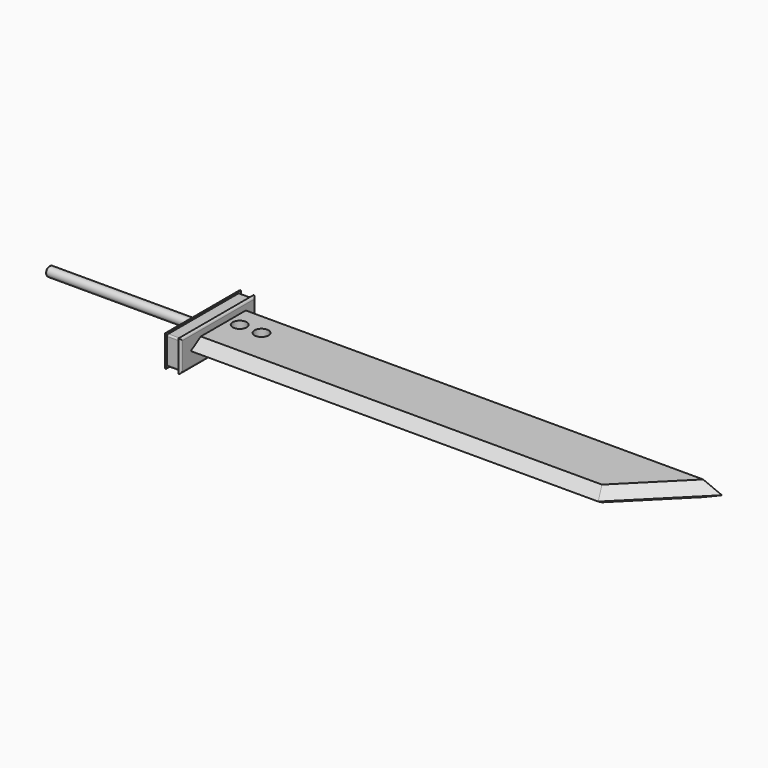
from build123d import *

# Parameters (mm, degrees)
F1_DEPTH    = 25
F2_T1_DEPTH = 1920.4823536212
F3_T1_DEPTH = 694.2958053538
F5_R        = 22.5
F6_DEPTH    = 100
F7_W        = 55
F7_H        = 300
F8_DEPTH    = 50
F9_R        = 7
F10_DEPTH   = 5
F11_DEPTH   = 5
F12_DEPTH   = 5
F13_DEPTH   = 5
F14_R       = 5
F15_W       = 500
F15_H       = 15
F17_R       = 5
F18_R       = 5


# Not quite as in the source:
# - a fillet or chamfer that OpenCascade refuses, or shapes differently, is made with other operations: its cross-section is extruded or revolved along the edge and cut away or added
# - a feature names something its author has since deleted; it is built from what else it names


with BuildPart() as f1:
    # F0 (on Top) → F1 (new body)
    with BuildSketch(Plane.XY):
        Polygon((1600, 0), (0, 0), (0, -300), (1300, -300), align=None)
    extrude(amount=F1_DEPTH)

    # F2: chamfer of 120 x 75 on 1 edges, made by hand

    # F2_s2 → F2_t1 (cut)
    with BuildSketch(Plane.YZ.offset(-310.2411768106)):
        Polygon((-300, -50), (-180, 25), (-300, 25), align=None)
    extrude(amount=F2_T1_DEPTH, mode=Mode.SUBTRACT)

    # F3: chamfer of 50 x 85 on 1 edges, made by hand

    # F3_s2 → F3_t1 (cut)
    with BuildSketch(Plane(origin=(464.5293639425, 464.5293639425, 0), x_dir=(0, 0, 1), z_dir=(0.7071067812, 0.7071067812, 0))):
        Polygon((-25, 1131.3708498985), (25, 1046.3708498985), (25, 1131.3708498985), align=None)
    extrude(amount=F3_T1_DEPTH, mode=Mode.SUBTRACT)

    # F4: F1 across face


with BuildPart() as f1_1:
    add(f1.part)
    add(f1.part.mirror(Plane(origin=(716.3583208568, -107.1792818856, 0), x_dir=(1, 0, 0), z_dir=(0, 0, -1))))

    # F5 (on face) → F6 (cut)
    with BuildSketch(Plane.XY.offset(25)):
        with Locations((52, -70)):
            Circle(F5_R)
        with Locations((122, -70)):
            Circle(F5_R)
    extrude(amount=-F6_DEPTH, mode=Mode.SUBTRACT)


with BuildPart() as f8:
    # F7 (on Top) → F8 (new body, symmetric)
    with BuildSketch(Plane.XY):
        with Locations((-11.9931862531, -110)):
            Rectangle(F7_W, F7_H)
    extrude(amount=F8_DEPTH, both=True)

    # F9
    f9_edges = [f8.edges().sort_by_distance(p)[0] for p in [
        (15.506814, -110, 50),
        (15.506814, -110, -50),
        (-39.493186, -110, 50),
        (-39.493186, -260, 0),
        (-39.493186, -110, -50),
        (-39.493186, 40, 0),
        (15.506814, -260, 0),
        (15.506814, 40, 0),
    ]]
    fillet(f9_edges, radius=F9_R)

    # F10 (cut): a face of the model
    f10_faces = [f8.faces().sort_by_distance(p)[0] for p in [
        (-11.9931862531, -110, 50),
    ]]
    extrude(f10_faces, amount=-F10_DEPTH, mode=Mode.SUBTRACT)

    # F11 (cut): a face of the model
    f11_faces = [f8.faces().sort_by_distance(p)[0] for p in [
        (-11.9931862531, -260, -2.5),
    ]]
    extrude(f11_faces, amount=-F11_DEPTH, mode=Mode.SUBTRACT)

    # F12 (cut): a face of the model
    f12_faces = [f8.faces().sort_by_distance(p)[0] for p in [
        (-11.9931862531, -107.5, -50),
    ]]
    extrude(f12_faces, amount=-F12_DEPTH, mode=Mode.SUBTRACT)

    # F13 (cut): a face of the model
    f13_faces = [f8.faces().sort_by_distance(p)[0] for p in [
        (-11.9931862531, 40, 0),
    ]]
    extrude(f13_faces, amount=-F13_DEPTH, mode=Mode.SUBTRACT)

    # F14
    f14_edges = [f8.edges().sort_by_distance(p)[0] for p in [
        (-11.993186, -255, 45),
        (-11.993186, -255, -45),
        (-11.993186, 35, -45),
        (-11.993186, 35, 45),
    ]]
    fillet(f14_edges, radius=F14_R)

    # F15 (on Top) → F16 (revolve)
    with BuildSketch(Plane.XY):
        with Locations((-282.4931862531, -110.0347492099)):
            Rectangle(F15_W, F15_H)
    revolve(axis=Axis((-282.4931862531, -102.5347492099, 0), (1, 0, 0)))

    # F17
    f17_edges = [f8.edges().sort_by_distance(p)[0] for p in [
        (-532.493186, -87.534749, 0),
    ]]
    fillet(f17_edges, radius=F17_R)

    # F18
    f18_edges = [f8.edges().sort_by_distance(p)[0] for p in [
        (-39.493186, -87.534749, 0),
    ]]
    fillet(f18_edges, radius=F18_R)

    # F19: cut F1
    add(f1_1.part, mode=Mode.SUBTRACT)


solid = Compound([f1_1.part, f8.part])
